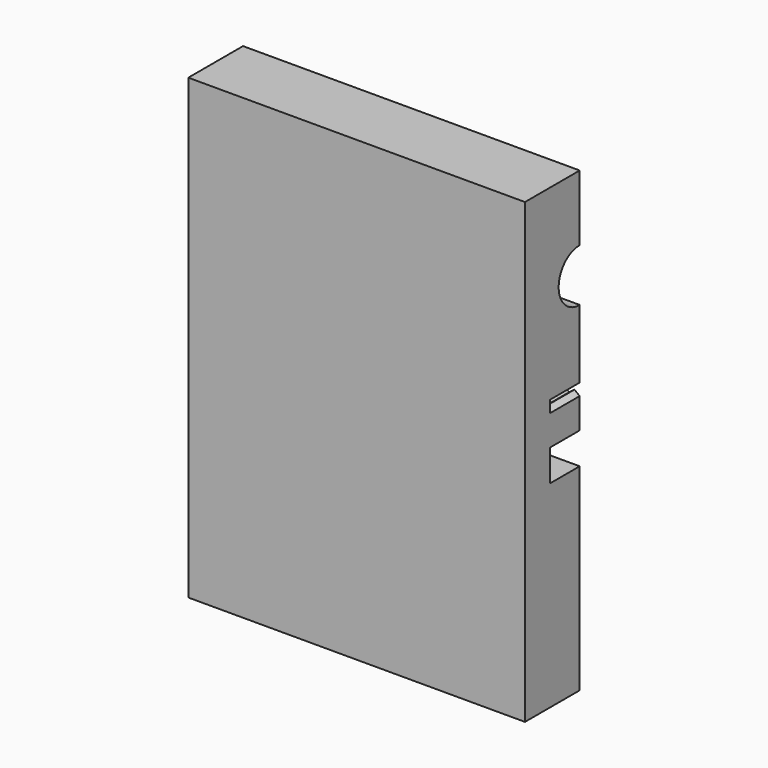
from build123d import *

# Parameters (mm, degrees)
F0_W      = 64
F0_H      = 87
F1_DEPTH  = 13
F3_DEPTH  = 7
F5_DEPTH  = 29.5
F7_DEPTH  = 29.5
F9_DEPTH  = 5
F10_DEPTH = 5
F12_DEPTH = 64.001


with BuildPart() as f1:
    # F0 (on Front) → F1 (new body)
    with BuildSketch(Plane.XZ):
        with Locations((1.2601554287, 25.9569030584)):
            Rectangle(F0_W, F0_H)
    extrude(amount=-F1_DEPTH)

    # F2 (on face) → F3 (cut)
    with BuildSketch(Plane(origin=(0, 13, 0), x_dir=(-1, 0, 0), z_dir=(0, 1, 0))):
        Polygon((-11.2601554287, 33.9569030584), (-33.2601554287, 33.9569030584), (-33.2601554287, 31.7069030584), (-32.2601554287, 32.4569030584), (-31.2601554287, 31.7069030584), (-30.2601554287, 32.4569030584), (-29.2601554287, 31.7069030584), (-28.2601554287, 32.4569030584), (-27.2601554287, 31.7069030584), (-26.2601554287, 32.4569030584), (-25.2601554287, 31.7069030584), (-24.2601554287, 32.4569030584), (-23.2601554287, 31.7069030584), (-22.2601554287, 32.4569030584), (-21.2601554287, 31.7069030584), (-20.2601554287, 32.4569030584), (-19.2601554287, 31.7069030584), (-18.2601554287, 32.4569030584), (-17.2601554287, 31.7069030584), (-16.2601554287, 32.4569030584), (-15.2601554287, 31.7069030584), (-14.2601554287, 32.4569030584), (-13.2601554287, 31.7069030584), (-12.2601554287, 32.4569030584), (-11.2601554287, 31.7069030584), align=None)
        Polygon((8.7398445713, 33.9569030584), (-11.2601554287, 33.9569030584), (-11.2601554287, 31.7069030584), (-10.2601554287, 32.4569030584), (-9.2601554287, 31.7069030584), (-8.2601554287, 32.4569030584), (-7.2601554287, 31.7069030584), (-6.2601554287, 32.4569030584), (-5.2601554287, 31.7069030584), (-4.2601554287, 32.4569030584), (-3.2601554287, 31.7069030584), (-2.2601554287, 32.4569030584), (-1.2601554287, 31.7069030584), (-0.2601554287, 32.4569030584), (0.7398445713, 31.7069030584), (1.7398445713, 32.4569030584), (2.7398445713, 31.7069030584), (3.7398445713, 32.4569030584), (4.7398445713, 31.7069030584), (5.7398445713, 32.4569030584), (6.7398445713, 31.7069030584), (7.7398445713, 32.4569030584), (8.7398445713, 31.7069030584), align=None)
        Polygon((-9.2601554287, 31.7069030584), (-11.2601554287, 31.7069030584), (-11.2601554287, 25.9569030584), (8.7398445713, 25.9569030584), (8.7398445713, 31.7069030584), (6.7398445713, 31.7069030584), (4.7398445713, 31.7069030584), (2.7398445713, 31.7069030584), (0.7398445713, 31.7069030584), (-1.2601554287, 31.7069030584), (-3.2601554287, 31.7069030584), (-5.2601554287, 31.7069030584), (-7.2601554287, 31.7069030584), align=None)
        Polygon((30.7398445713, 33.9569030584), (8.7398445713, 33.9569030584), (8.7398445713, 31.7069030584), (9.7398445713, 32.4569030584), (10.7398445713, 31.7069030584), (11.7398445713, 32.4569030584), (12.7398445713, 31.7069030584), (13.7398445713, 32.4569030584), (14.7398445713, 31.7069030584), (15.7398445713, 32.4569030584), (16.7398445713, 31.7069030584), (17.7398445713, 32.4569030584), (18.7398445713, 31.7069030584), (19.7398445713, 32.4569030584), (20.7398445713, 31.7069030584), (21.7398445713, 32.4569030584), (22.7398445713, 31.7069030584), (23.7398445713, 32.4569030584), (24.7398445713, 31.7069030584), (25.7398445713, 32.4569030584), (26.7398445713, 31.7069030584), (27.7398445713, 32.4569030584), (28.7398445713, 31.7069030584), (29.7398445713, 32.4569030584), (30.7398445713, 31.7069030584), align=None)
        Polygon((-11.2601554287, 25.9569030584), (-33.2601554287, 25.9569030584), (-33.2601554287, 19.9569030584), (30.7398445713, 19.9569030584), (30.7398445713, 25.9569030584), (8.7398445713, 25.9569030584), align=None)
        Polygon((6.7398445713, 31.7069030584), (8.7398445713, 31.7069030584), (7.7398445713, 32.4569030584), align=None)
        Polygon((4.7398445713, 31.7069030584), (6.7398445713, 31.7069030584), (5.7398445713, 32.4569030584), align=None)
        Polygon((2.7398445713, 31.7069030584), (4.7398445713, 31.7069030584), (3.7398445713, 32.4569030584), align=None)
        Polygon((0.7398445713, 31.7069030584), (2.7398445713, 31.7069030584), (1.7398445713, 32.4569030584), align=None)
        Polygon((-1.2601554287, 31.7069030584), (0.7398445713, 31.7069030584), (-0.2601554287, 32.4569030584), align=None)
        Polygon((-2.2601554287, 32.4569030584), (-3.2601554287, 31.7069030584), (-1.2601554287, 31.7069030584), align=None)
        Polygon((-6.2601554287, 32.4569030584), (-7.2601554287, 31.7069030584), (-5.2601554287, 31.7069030584), align=None)
        Polygon((-4.2601554287, 32.4569030584), (-5.2601554287, 31.7069030584), (-3.2601554287, 31.7069030584), align=None)
        Polygon((-8.2601554287, 32.4569030584), (-9.2601554287, 31.7069030584), (-7.2601554287, 31.7069030584), align=None)
        Polygon((-10.2601554287, 32.4569030584), (-11.2601554287, 31.7069030584), (-9.2601554287, 31.7069030584), align=None)
    extrude(amount=-F3_DEPTH, mode=Mode.SUBTRACT)

    # F4 (on face) → F5 (cut, through all)
    with BuildSketch(Plane(origin=(-30.7398445713, 0, 0), x_dir=(0, -1, 0), z_dir=(-1, 0, 0))):
        with BuildLine():
            ThreePointArc((-13, 44.4569030584), (-7.6966991411, 46.6536021995), (-5.5, 51.9569030584))
            ThreePointArc((-5.5, 51.9569030584), (-7.6966991411, 57.2602039173), (-13, 59.4569030584))
            Line((-13, 59.4569030584), (-13, 44.4569030584))
        make_face()
    extrude(amount=-F5_DEPTH, mode=Mode.SUBTRACT)

    # F6 (on face) → F7 (cut, through all)
    with BuildSketch(Plane.YZ.offset(33.2601554287)):
        with BuildLine():
            Line((13, 44.2069030584), (13, 59.2069030584))
            ThreePointArc((13, 59.2069030584), (5.5, 51.7069030584), (13, 44.2069030584))
        make_face()
    extrude(amount=-F7_DEPTH, mode=Mode.SUBTRACT)

    # F8 (on face) → F9 (join)
    with BuildSketch(Plane.YZ.offset(33.2601554287)):
        with BuildLine():
            Line((13, 59.2069030584), (13, 64.3319030584))
            Line((13, 64.3319030584), (0, 64.3319030584))
            Line((0, 64.3319030584), (0, 38.0137264729))
            Line((0, 38.0137264729), (13, 38.0137264729))
            Line((13, 38.0137264729), (13, 44.2069030584))
            ThreePointArc((13, 44.2069030584), (5.5, 51.7069030584), (13, 59.2069030584))
        make_face()
        with BuildLine():
            Line((13, 44.2069030584), (13, 59.2069030584))
            ThreePointArc((13, 59.2069030584), (5.5, 51.7069030584), (13, 44.2069030584))
        make_face()
    extrude(amount=-F9_DEPTH)

    # F4 (on face) → F10 (join)
    with BuildSketch(Plane(origin=(-30.7398445713, 0, 0), x_dir=(0, -1, 0), z_dir=(-1, 0, 0))):
        with BuildLine():
            ThreePointArc((-13, 44.4569030584), (-7.6966991411, 46.6536021995), (-5.5, 51.9569030584))
            ThreePointArc((-5.5, 51.9569030584), (-7.6966991411, 57.2602039173), (-13, 59.4569030584))
            Line((-13, 59.4569030584), (-13, 44.4569030584))
        make_face()
    extrude(amount=-F10_DEPTH)

    # F11 (on face) → F12 (cut, through all)
    with BuildSketch(Plane(origin=(-30.7398445713, 0, 0), x_dir=(0, -1, 0), z_dir=(-1, 0, 0))):
        with BuildLine():
            ThreePointArc((-13, 46.9569030584), (-9.4644660941, 48.4213691524), (-8, 51.9569030584))
            ThreePointArc((-8, 51.9569030584), (-9.4644660941, 55.4924369643), (-13, 56.9569030584))
            Line((-13, 56.9569030584), (-13, 46.9569030584))
        make_face()
    extrude(amount=-F12_DEPTH, mode=Mode.SUBTRACT)


solid = f1.part
